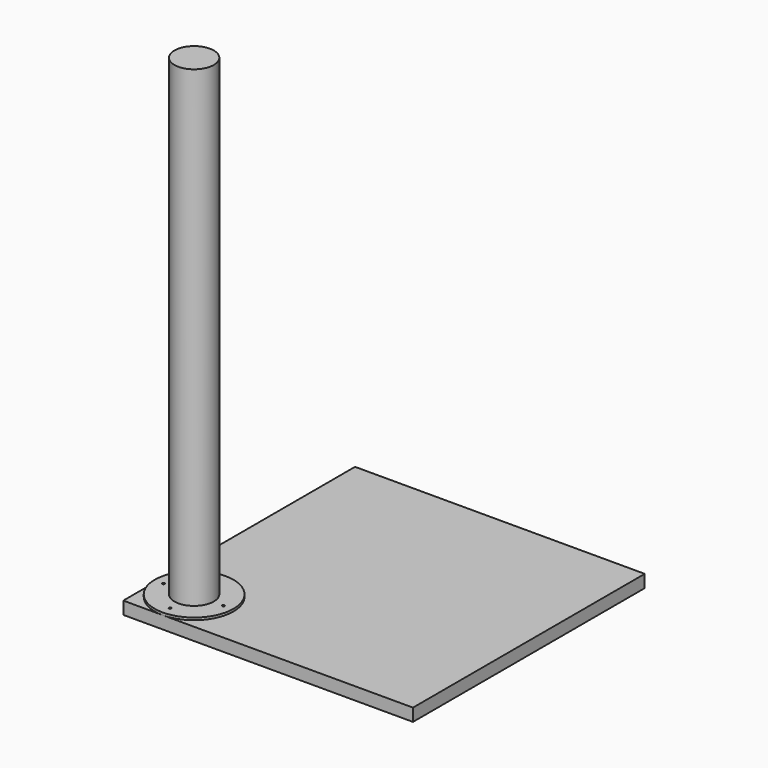
from build123d import *

# Parameters (mm, degrees)
F0_W     = 368
F0_H     = 368
F1_DEPTH = 16
F3_D     = 50
F3_DEPTH = 16
F3_TIP   = 15.0215154757
F2_R     = 50
F4_DEPTH = 3
F7_R     = 25
F8_DEPTH = 600
F9_D     = 3
F9_DEPTH = 3
F9_TIP   = 0.9012909285


# Not quite as in the source:
# - the program builds the solid bodies; features that only make, move or delete a surface that nothing else refers to are left out


with BuildPart() as f1:
    # F0 (on Top) → F1 (new body)
    with BuildSketch(Plane.XY):
        Rectangle(F0_W, F0_H)
    extrude(amount=F1_DEPTH)

    # F3
    with Locations(Plane.XY.offset(16)):
        with Locations((-134, -134)):
            Hole(F3_D / 2, depth=F3_DEPTH)
            with Locations((0, 0, -(F3_DEPTH + F3_TIP / 2))):  # 118° drill point
                Cone(0, F3_D / 2, F3_TIP, mode=Mode.SUBTRACT)

    # F2 (on face) → F4 (join)
    with BuildSketch(Plane.XY.offset(16)):
        with Locations((-134, -134)):
            Circle(F2_R)
    extrude(amount=F4_DEPTH)

    # F7 (on face) → F8 (join)
    with BuildSketch(Plane.XY.offset(19)):
        with Locations((-134, -134)):
            Circle(F7_R)
    extrude(amount=F8_DEPTH)

    # F9 (one way)
    with BuildSketch(Plane(origin=(0, 0, 16), x_dir=(1, 0, 0), z_dir=(0, 0, -1))):
        with Locations((-134, 96), (-171.9844305378, 135.0876749154), (-96.0155694622, 135.0876749154), (-134, 172)):
            Circle(F9_D / 2)
    extrude(amount=-F9_DEPTH, mode=Mode.SUBTRACT)
    with Locations(Plane(origin=(0, 0, 16), x_dir=(1, 0, 0), z_dir=(0, 0, -1))):
        with Locations((-134, 96), (-171.9844305378, 135.0876749154), (-96.0155694622, 135.0876749154), (-134, 172)):
            with Locations((0, 0, -(F9_DEPTH + F9_TIP / 2))):  # 118° drill point
                Cone(0, F9_D / 2, F9_TIP, mode=Mode.SUBTRACT)


solid = f1.part
